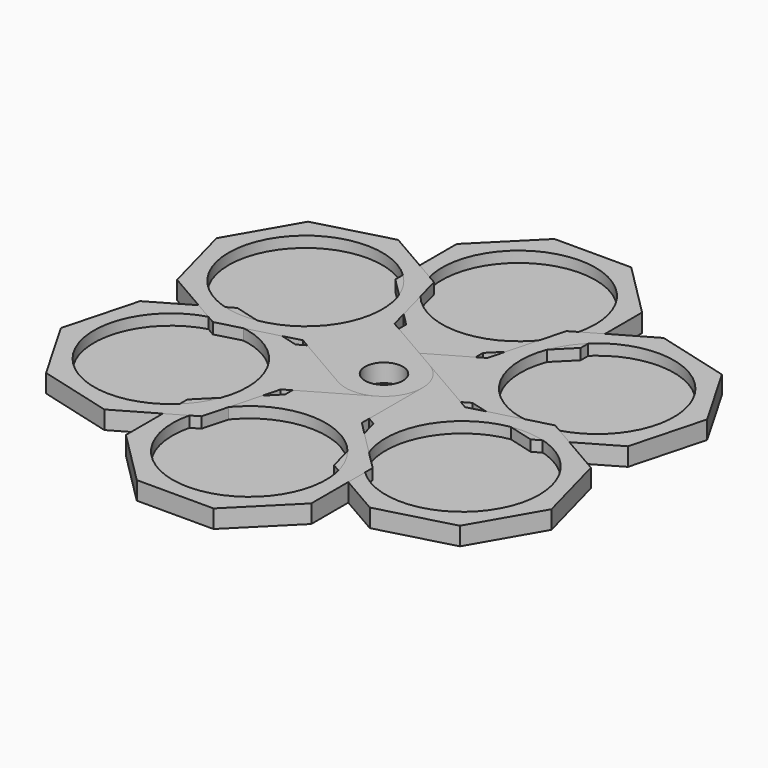
from build123d import *

# Parameters (mm, degrees)
F1_R     = 3.1369
F1_R_2   = 12.6913363088
F2_DEPTH = 3
F3_COUNT = 6
F5_R     = 14.6670401364
F6_DEPTH = 1.2
F7_COUNT = 6
F8_R     = 3.1369
F9_DEPTH = 25.4


# Not quite as in the source:
# - ends of sketch curves that miss each other by under 0.0002 mm in the source are joined
# - a feature names something its author has since deleted; it is built from what else it names


with BuildPart() as f2:
    # F1 (on Top) → F2 (new body)
    with BuildSketch(Plane.XY):
        with BuildLine():
            Line((-6.3474243933, 12.5191587118), (-6.3499997312, 0.0013064058))
            ThreePointArc((-6.3499997312, 0.0013064058), (-6.3499999664, 0.0006532029), (-6.35, 0))
            ThreePointArc((-6.35, 0), (-0.0904298143, -6.3493560657), (6.3474243933, -0.1808412882))
            Line((6.3474243933, -0.1808412882), (6.3474243933, 0.1808412882))
            Line((6.3474243933, 0.1808412882), (6.3474243933, 12.5191587118))
            Line((6.3474243933, 12.5191587118), (15.3240380564, 21.4957723749))
            Line((15.3240380564, 21.4957723749), (15.3240380564, 34.1906211614))
            Line((15.3240380564, 34.1906211614), (6.3474243933, 43.1672348246))
            Line((6.3474243933, 43.1672348246), (-6.3474243933, 43.1672348246))
            Line((-6.3474243933, 43.1672348246), (-15.3240380564, 34.1906211614))
            Line((-15.3240380564, 34.1906211614), (-15.3240380564, 21.4957723749))
            Line((-15.3240380564, 21.4957723749), (-6.3474243933, 12.5191587118))
        make_face()
        Circle(F1_R, mode=Mode.SUBTRACT)
        with Locations((0, 27.8431967682)):
            Circle(F1_R_2, mode=Mode.SUBTRACT)
        Circle(F1_R)
    extrude(amount=F2_DEPTH)


with BuildPart() as f3_1:
    # F3: instance of F2
    add(f2.part.rotate(Axis((0, 0, -15.3654031456), (0, 0, -1)), 1 * 360 / F3_COUNT))


with BuildPart() as f3_2:
    # F3: instance of F2
    add(f2.part.rotate(Axis((0, 0, -15.3654031456), (0, 0, -1)), 2 * 360 / F3_COUNT))


with BuildPart() as f3_3:
    # F3: instance of F2
    add(f2.part.rotate(Axis((0, 0, -15.3654031456), (0, 0, -1)), 3 * 360 / F3_COUNT))


with BuildPart() as f3_4:
    # F3: instance of F2
    add(f2.part.rotate(Axis((0, 0, -15.3654031456), (0, 0, -1)), 4 * 360 / F3_COUNT))


with BuildPart() as f3_5:
    # F3: instance of F2
    add(f2.part.rotate(Axis((0, 0, -15.3654031456), (0, 0, -1)), 5 * 360 / F3_COUNT))


with BuildPart() as f6:
    # F5 (on Top) → F6 (new body)
    with BuildSketch(Plane.XY):
        with Locations((0, 27.6992823929)):
            Circle(F5_R)
    extrude(amount=F6_DEPTH)


with BuildPart() as f7_1:
    # F7: instance of F6
    add(f6.part.rotate(Axis((0, 0, -11.0484389588), (0, 0, -1)), 1 * 360 / F7_COUNT))


with BuildPart() as f7_2:
    # F7: instance of F6
    add(f6.part.rotate(Axis((0, 0, -11.0484389588), (0, 0, -1)), 2 * 360 / F7_COUNT))


with BuildPart() as f7_3:
    # F7: instance of F6
    add(f6.part.rotate(Axis((0, 0, -11.0484389588), (0, 0, -1)), 3 * 360 / F7_COUNT))


with BuildPart() as f7_4:
    # F7: instance of F6
    add(f6.part.rotate(Axis((0, 0, -11.0484389588), (0, 0, -1)), 4 * 360 / F7_COUNT))


with BuildPart() as f7_5:
    # F7: instance of F6
    add(f6.part.rotate(Axis((0, 0, -11.0484389588), (0, 0, -1)), 5 * 360 / F7_COUNT))


with BuildPart() as f9_tool:
    # F8 (on Top) → F9 (new body)
    with BuildSketch(Plane.XY):
        Circle(F8_R)
    extrude(amount=F9_DEPTH)


with BuildPart() as f2_1:
    add(f2.part)

    # F9: cut by f9_tool
    add(f9_tool.part, mode=Mode.SUBTRACT)


with BuildPart() as f3_1_1:
    add(f3_1.part)

    # F9: cut by f9_tool
    add(f9_tool.part, mode=Mode.SUBTRACT)


with BuildPart() as f3_2_1:
    add(f3_2.part)

    # F9: cut by f9_tool
    add(f9_tool.part, mode=Mode.SUBTRACT)


with BuildPart() as f3_3_1:
    add(f3_3.part)

    # F9: cut by f9_tool
    add(f9_tool.part, mode=Mode.SUBTRACT)


with BuildPart() as f3_4_1:
    add(f3_4.part)

    # F9: cut by f9_tool
    add(f9_tool.part, mode=Mode.SUBTRACT)


with BuildPart() as f3_5_1:
    add(f3_5.part)

    # F9: cut by f9_tool
    add(f9_tool.part, mode=Mode.SUBTRACT)


solid = Compound([f6.part, f7_1.part, f7_2.part, f7_3.part, f7_4.part, f7_5.part, f2_1.part, f3_1_1.part, f3_2_1.part, f3_3_1.part, f3_4_1.part, f3_5_1.part])
